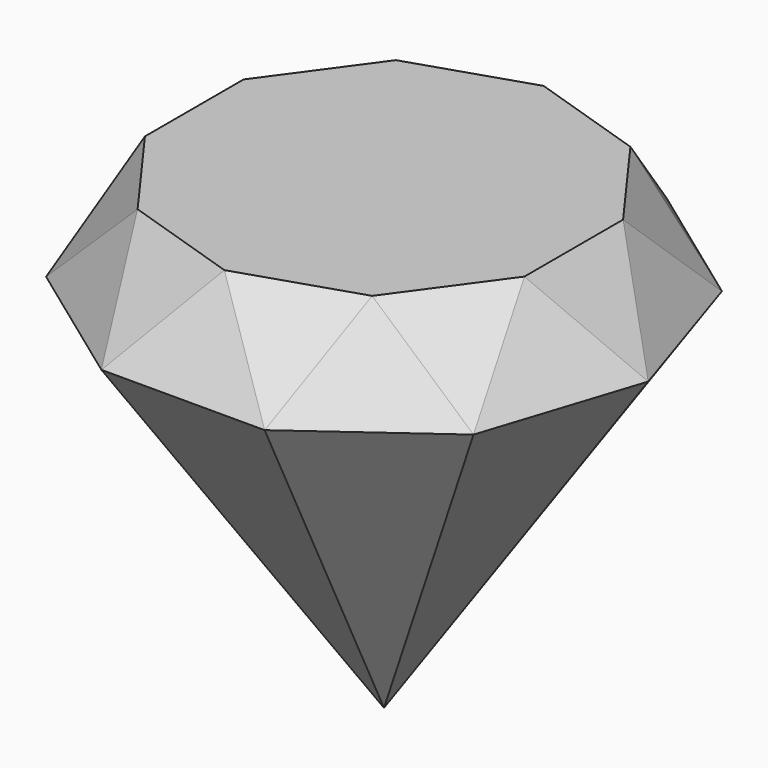
from build123d import *

# Parameters (mm, degrees)
F5_DEPTH        = 20
F5_TAPER        = 29
F8_COPIES_COUNT = 10


# Not quite as in the source:
# - a pattern or mirror of a feature is missing from the dataset's text; its kind, count and spacing are read off the source's solid


with BuildPart() as f3:
    # F1 (on offset) → F3 section 0
    with BuildSketch(Plane.XY.offset(80), mode=Mode.PRIVATE) as f3_s0:
        Polygon((45.8155948031, -33.2869780703), (56.6311896062, 0), (45.8155948031, 33.2869780703), (17.5, 53.8594619006), (-17.5, 53.8594619006), (-45.8155948031, 33.2869780703), (-56.6311896062, 0), (-45.8155948031, -33.2869780703), (-17.5, -53.8594619006), (17.5, -53.8594619006), align=None)
    loft([Vertex(0, 0, 0), f3_s0.sketch])

    # F4 (on face) → F5 (join)
    with BuildSketch(Plane.XY.offset(80)):
        Polygon((45.8155948031, -33.2869780703), (56.6311896062, 0), (45.8155948031, 33.2869780703), (17.5, 53.8594619006), (-17.5, 53.8594619006), (-45.8155948031, 33.2869780703), (-56.6311896062, 0), (-45.8155948031, -33.2869780703), (-17.5, -53.8594619006), (17.5, -53.8594619006), align=None)
    extrude(amount=F5_DEPTH, taper=F5_TAPER)

    # F6 (on face) → F8 section 0
    with BuildSketch(Plane.XY.offset(100), mode=Mode.PRIVATE) as f8_s0:
        Polygon((44.9744890431, 0), (40.6798074962, 13.2176706945), (40.6798074962, -13.2176706945), align=None)
    f8 = loft([f8_s0.sketch, Vertex(56.6311896062, 0, 80)], mode=Mode.SUBTRACT)

    # F8_copies: F8 ×10 about axis
    f8_copies_axis = Axis((0, 0, 0), (0, 0, 1))
    for i in range(1, F8_COPIES_COUNT):
        add(f8.rotate(f8_copies_axis, i * 360 / F8_COPIES_COUNT), mode=Mode.SUBTRACT)


solid = f3.part
